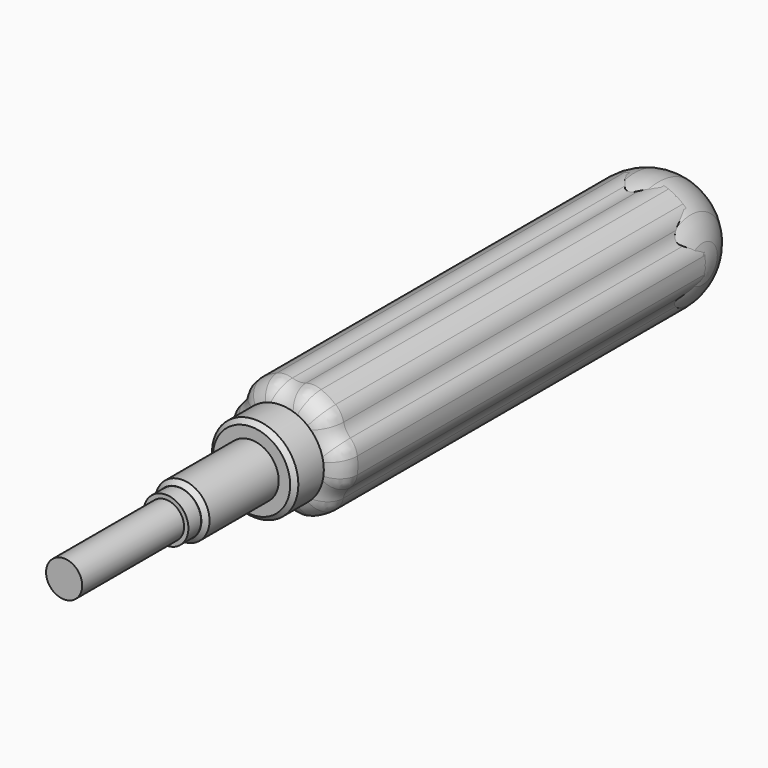
from build123d import *

# Parameters (mm, degrees)
F0_R      = 3.975
F1_DEPTH  = 28
F2_R      = 4.925
F3_DEPTH  = 3.5
F4_R      = 5.975
F5_DEPTH  = 128.5
F6_SIZE2  = 1
F6_SIZE   = 1
F7_R      = 4.975
F8_DEPTH  = 100.5
F9_R      = 9.5
F10_DEPTH = 8
F11_SIZE  = 1
F14_R     = 5
F15_F1_R  = 5
F15_F2_R  = 5
F15_F3_R  = 5
F15_F4_R  = 5
F15_F5_R  = 5
F15_F6_R  = 5
F15_F7_R  = 4.9996


# Not quite as in the source:
# - a fillet or chamfer is up to 0.001 mm smaller than in the source, because OpenCascade refuses the exact size


with BuildPart() as f1:
    # F0 (on Front) → F1 (new body)
    with BuildSketch(Plane.XZ):
        Circle(F0_R)
    extrude(amount=-F1_DEPTH)

    # F2 (on face) → F3 (join)
    with BuildSketch(Plane(origin=(0, 28, 0), x_dir=(-1, 0, 0), z_dir=(0, 1, 0))):
        Circle(F2_R)
    extrude(amount=F3_DEPTH)

    # F4 (on face) → F5 (join)
    with BuildSketch(Plane(origin=(0, 31.5, 0), x_dir=(-1, 0, 0), z_dir=(0, 1, 0))):
        Circle(F4_R)
    extrude(amount=F5_DEPTH)

    # F6
    f6_edges = [f1.edges().sort_by_distance(p)[0] for p in [
        (-5.975, 95.75, 0),
        (5.975, 31.5, 0),
        (5.975, 160, 0),
    ]]
    chamfer(f6_edges, length=F6_SIZE, length2=F6_SIZE2)


with BuildPart() as f8:
    # F7 (on face) → F8 (new body)
    with BuildSketch(Plane(origin=(0, 160, 0), x_dir=(-1, 0, 0), z_dir=(0, 1, 0))):
        with BuildLine():
            ThreePointArc((12.3687487082, -4.0017565384), (12.8412174891, -2.0256192625), (13, 0))
            ThreePointArc((13, 0), (12.8293602369, 2.0994084671), (12.321920629, 4.1437026936))
            ThreePointArc((12.321920629, 4.1437026936), (10.3323229846, 6.0448336313), (9.6499971762, 8.7107723251))
            ThreePointArc((9.6499971762, 8.7107723251), (6.4351697459, 11.2955119557), (2.5724085161, 12.7429476349))
            ThreePointArc((2.5724085161, 12.7429476349), (-0.068817994, 11.9704710004), (-2.7187515321, 12.7125288636))
            ThreePointArc((-2.7187515321, 12.7125288636), (-6.5646154294, 11.2207764555), (-9.7495121129, 8.5992449413))
            ThreePointArc((-9.7495121129, 8.5992449413), (-10.4011409786, 5.9256373692), (-12.3687487082, 4.0017565384))
            ThreePointArc((-12.3687487082, 4.0017565384), (-12.9997851753, -0.0747355002), (-12.321920629, -4.1437026936))
            ThreePointArc((-12.321920629, -4.1437026936), (-10.3323229846, -6.0448336313), (-9.6499971762, -8.7107723251))
            ThreePointArc((-9.6499971762, -8.7107723251), (-6.4351697459, -11.2955119557), (-2.5724085161, -12.7429476349))
            ThreePointArc((-2.5724085161, -12.7429476349), (0.068817994, -11.9704710004), (2.7187515321, -12.7125288636))
            ThreePointArc((2.7187515321, -12.7125288636), (6.5646154294, -11.2207764555), (9.7495121129, -8.5992449413))
            ThreePointArc((9.7495121129, -8.5992449413), (10.4011409786, -5.9256373692), (12.3687487082, -4.0017565384))
        make_face()
        Circle(F7_R, mode=Mode.SUBTRACT)
    extrude(amount=-F8_DEPTH)

    # F14
    f14_edges = [f8.edges().sort_by_distance(p)[0] for p in [
        (-12.368749, 109.75, -4.001757),
        (-9.649997, 109.75, 8.710772),
        (2.718752, 109.75, 12.712529),
        (12.368749, 109.75, 4.001757),
        (9.649997, 109.75, -8.710772),
        (-2.718752, 109.75, -12.712529),
    ]]
    fillet(f14_edges, radius=F14_R)

    # F15: fillet of radius 5 on 10 edges, made by hand

    # F15_f1
    f15_f1_edges = [f8.edges().sort_by_distance(p)[0] for p in [
        (-12.321920629, 109.75, 4.1437026936),
    ]]
    fillet(f15_f1_edges, radius=F15_F1_R)

    # F15_f2
    f15_f2_edges = [f8.edges().sort_by_distance(p)[0] for p in [
        (-9.7495121129, 109.75, -8.5992449413),
    ]]
    fillet(f15_f2_edges, radius=F15_F2_R)

    # F15_f3
    f15_f3_edges = [f8.edges().sort_by_distance(p)[0] for p in [
        (-2.5724085161, 109.75, 12.7429476349),
    ]]
    fillet(f15_f3_edges, radius=F15_F3_R)

    # F15_f4
    f15_f4_edges = [f8.edges().sort_by_distance(p)[0] for p in [
        (2.5724085161, 109.75, -12.7429476349),
    ]]
    fillet(f15_f4_edges, radius=F15_F4_R)

    # F15_f5
    f15_f5_edges = [f8.edges().sort_by_distance(p)[0] for p in [
        (9.7495121129, 109.75, 8.5992449413),
    ]]
    fillet(f15_f5_edges, radius=F15_F5_R)

    # F15_f6
    f15_f6_edges = [f8.edges().sort_by_distance(p)[0] for p in [
        (12.321920629, 109.75, -4.1437026936),
    ]]
    fillet(f15_f6_edges, radius=F15_F6_R)

    # F15_f7 (radius 5 in the source; OpenCascade refuses exactly that, so slightly less here)
    f15_f7_edges = [f8.edges().sort_by_distance(p)[0] for p in [
        (-10.3323229846, 59.5, 6.0448336313),
        (-9.1167477681, 59.5, 9.0139426757),
        (-6.4351697459, 59.5, 11.2955119557),
    ]]
    fillet(f15_f7_edges, radius=F15_F7_R)


with BuildPart() as f10:
    # F9 (on face) → F10 (new body)
    with BuildSketch(Plane.XZ.offset(-59.5)):
        Circle(F9_R)
    extrude(amount=F10_DEPTH)

    # F11
    f11_edges = [f10.edges().sort_by_distance(p)[0] for p in [
        (-9.5, 51.5, 0),
    ]]
    chamfer(f11_edges, length=F11_SIZE)


with BuildPart() as f13:
    # F12 (on face) → F13 (revolve)
    with BuildSketch(Plane(origin=(0, 160, 0), x_dir=(-1, 0, 0), z_dir=(0, 1, 0))):
        with BuildLine():
            ThreePointArc((12.3687487082, -4.0017565384), (12.8412174891, -2.0256192625), (13, 0))
            ThreePointArc((13, 0), (12.9999462937, 0.0373679045), (12.9997851753, 0.0747355002))
            Line((12.9997851753, 0.0747355002), (4.9749177883, 0.0286007011))
            ThreePointArc((4.9749177883, 0.0286007011), (4.974979447, 0.0143004096), (4.975, 0))
            ThreePointArc((4.975, 0), (0.0143004096, -4.974979447), (-4.9749177883, -0.0286007011))
            Line((-4.9749177883, -0.0286007011), (-12.9997851753, -0.0747355002))
            ThreePointArc((-12.9997851753, -0.0747355002), (-12.8232725821, -2.1362772022), (-12.321920629, -4.1437026936))
            ThreePointArc((-12.321920629, -4.1437026936), (-10.3323229846, -6.0448336313), (-9.6499971762, -8.7107723251))
            ThreePointArc((-9.6499971762, -8.7107723251), (-6.4351697459, -11.2955119557), (-2.5724085161, -12.7429476349))
            ThreePointArc((-2.5724085161, -12.7429476349), (0.068817994, -11.9704710004), (2.7187515321, -12.7125288636))
            ThreePointArc((2.7187515321, -12.7125288636), (6.5646154294, -11.2207764555), (9.7495121129, -8.5992449413))
            ThreePointArc((9.7495121129, -8.5992449413), (10.4011409786, -5.9256373692), (12.3687487082, -4.0017565384))
        make_face()
        with BuildLine():
            ThreePointArc((9.7495121129, -8.5992449413), (11.2955119557, -6.4351697459), (12.3687487082, -4.0017565384))
            ThreePointArc((12.3687487082, -4.0017565384), (10.4011409786, -5.9256373692), (9.7495121129, -8.5992449413))
        make_face()
        with BuildLine():
            ThreePointArc((-2.5724085161, -12.7429476349), (0.0747355002, -12.9997851753), (2.7187515321, -12.7125288636))
            ThreePointArc((2.7187515321, -12.7125288636), (0.068817994, -11.9704710004), (-2.5724085161, -12.7429476349))
        make_face()
        with BuildLine():
            ThreePointArc((-9.6499971762, -8.7107723251), (-10.3323229846, -6.0448336313), (-12.321920629, -4.1437026936))
            ThreePointArc((-12.321920629, -4.1437026936), (-11.2207764555, -6.5646154294), (-9.6499971762, -8.7107723251))
        make_face()
    revolve(axis=Axis((0, 160, 0), (-0.999983475, 0, 0.0057488846)))


solid = Compound([f1.part, f8.part, f10.part, f13.part])
